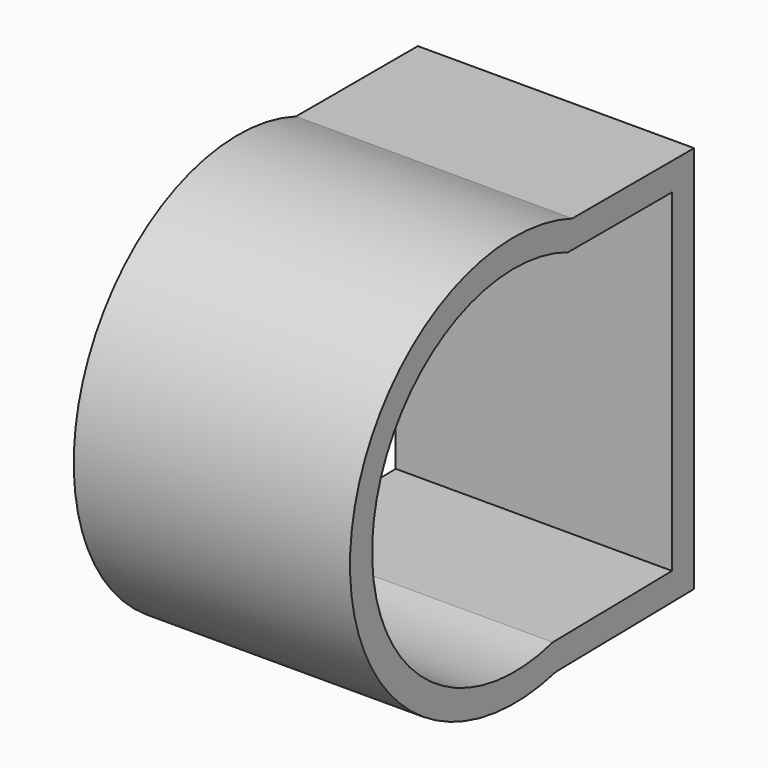
from build123d import *

# Parameters (mm, degrees)
F1_DEPTH = 30
F2_T     = 3


with BuildPart() as f1:
    # F0 (on Right) → F1 (new body)
    with BuildSketch(Plane.YZ):
        with BuildLine():
            ThreePointArc((-50.5638438315, 48.3802992553), (-77.1344876234, 31.6163385121), (-52.6412177761, 11.9412470637))
            Line((-52.6412177761, 11.9412470637), (-36.4591793272, 12.1873354573))
            Line((-36.4591793272, 12.1873354573), (-36.4591793272, 42.854900606))
            Line((-36.4591793272, 42.854900606), (-36.4591793272, 48.3802992553))
            Line((-36.4591793272, 48.3802992553), (-38.9720265736, 48.3802992553))
            Line((-38.9720265736, 48.3802992553), (-50.5638438315, 48.3802992553))
        make_face()
    extrude(amount=F1_DEPTH)

    # F2
    f2_openings = [f1.faces().sort_by_distance(p)[0] for p in [
        (30, -55.280278, 30.40174),
        (0, -55.280278, 30.40174),
    ]]
    offset(amount=F2_T, openings=f2_openings, kind=Kind.INTERSECTION)


solid = f1.part
